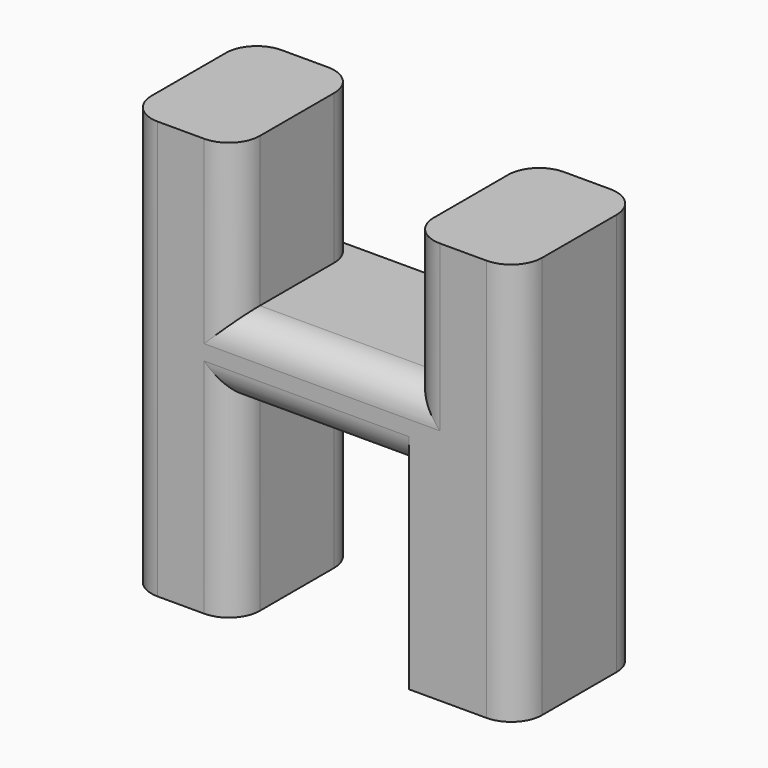
from build123d import *

# Parameters (mm, degrees)
F1_DEPTH = 12.7
F0_W     = 17.78
F0_H     = 2.54
F0_W_2   = 28.5250723219
F0_H_2   = 12.6543707534
F0_H_3   = 4.4012725921
F2_DEPTH = 25.4
F3_R     = 5.08


with BuildPart() as f1:
    # F0 (on Front) → F1 (new body)
    with BuildSketch(Plane.XZ):
        Polygon((8.89, 33.02), (-8.89, 33.02), (-8.89, -33.02), (8.89, -33.02), (8.89, -4.1522149311), (8.89, 8.5021558223), align=None)
    extrude(amount=F1_DEPTH)

    # F0 (on Front) → F2 (join)
    with BuildSketch(Plane.XZ):
        Polygon((8.89, 33.02), (-8.89, 33.02), (-8.89, -33.02), (8.89, -33.02), (8.89, -4.1522149311), (8.89, 8.5021558223), align=None)
        with Locations((0, -34.29)):
            Rectangle(F0_W, F0_H)
        with Locations((23.1525361609, 2.1749704456)):
            Rectangle(F0_W_2, F0_H_2)
        Polygon((37.4150723219, 30.48), (37.4150723219, 8.5021558223), (37.4150723219, -4.1522149311), (37.4150723219, -31.1587274079), (55.1950723219, -31.1587274079), (55.1950723219, 30.48), align=None)
        with Locations((46.3050723219, -33.359363704)):
            Rectangle(F0_W, F0_H_3)
    extrude(amount=F2_DEPTH)

    # F3
    f3_edges = [f1.edges().sort_by_distance(p)[0] for p in [
        (55.195072, -25.4, -2.54),
        (55.195072, 0, -2.54),
        (37.415072, -25.4, 19.491078),
        (8.89, -25.4, 20.761078),
        (8.89, -25.4, -19.856107),
        (-8.89, -25.4, -1.27),
        (23.152536, -25.4, 8.502156),
        (23.152536, -25.4, -4.152215),
        (37.415072, 0, -19.856107),
        (37.415072, 0, 19.491078),
        (23.152536, 0, -4.152215),
        (8.89, 0, 20.761078),
        (8.89, 0, -19.856107),
        (-8.89, 0, -1.27),
    ]]
    fillet(f3_edges, radius=F3_R)


solid = f1.part
